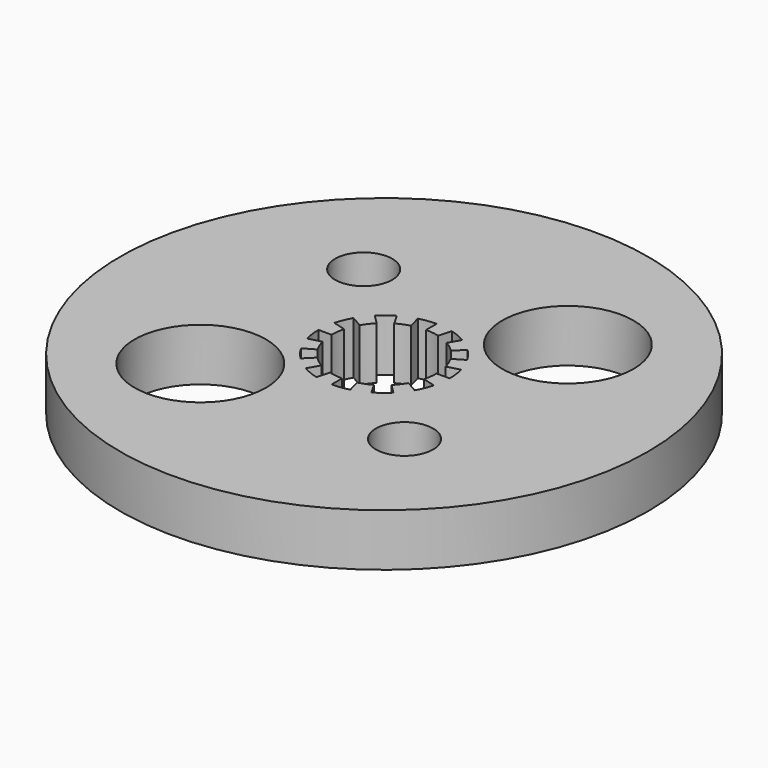
from build123d import *

# Parameters (mm, degrees)
F0_R            = 15.961960717
F0_R_2          = 3.96875
F0_R_3          = 3.175
F0_R_4          = 1.7272
F1_DEPTH        = 3.175
F3_DEPTH        = 3.175
F3_COPIES_COUNT = 12


# Not quite as in the source:
# - a pattern or mirror of a feature is missing from the dataset's text; its kind, count and spacing are read off the source's solid


with BuildPart() as f1:
    # F0 (on Top) → F1 (new body)
    with BuildSketch(Plane.XY):
        Circle(F0_R)
        with Locations((-6.1739260832, -6.1739260832)):
            Circle(F0_R_2, mode=Mode.SUBTRACT)
        Circle(F0_R_3, mode=Mode.SUBTRACT)
        with Locations((6.1739260832, -6.1739260832)):
            Circle(F0_R_4, mode=Mode.SUBTRACT)
        with Locations((-6.1739260832, 6.1739260832)):
            Circle(F0_R_4, mode=Mode.SUBTRACT)
        with Locations((6.1739260832, 6.1739260832)):
            Circle(F0_R_2, mode=Mode.SUBTRACT)
    extrude(amount=F1_DEPTH)

    # F2 (on face) → F3 (cut, through all)
    with BuildSketch(Plane.XY.offset(3.175)):
        with BuildLine():
            Line((-1.0271880853, 3.8335181231), (-0.8217504682, 3.0668144985))
            ThreePointArc((-0.8217504682, 3.0668144985), (-0.4144206603, 3.1478374349), (0, 3.175))
            Line((0, 3.175), (0, 3.96875))
            ThreePointArc((0, 3.96875), (-0.5180258254, 3.9347967936), (-1.0271880853, 3.8335181231))
        make_face()
    f3 = extrude(amount=-F3_DEPTH, mode=Mode.SUBTRACT)

    # F3_copies: F3 ×12 about axis
    f3_copies_axis = Axis((0, 0, 0), (0, 0, 1))
    for i in range(1, F3_COPIES_COUNT):
        add(f3.rotate(f3_copies_axis, i * 360 / F3_COPIES_COUNT), mode=Mode.SUBTRACT)


solid = f1.part
